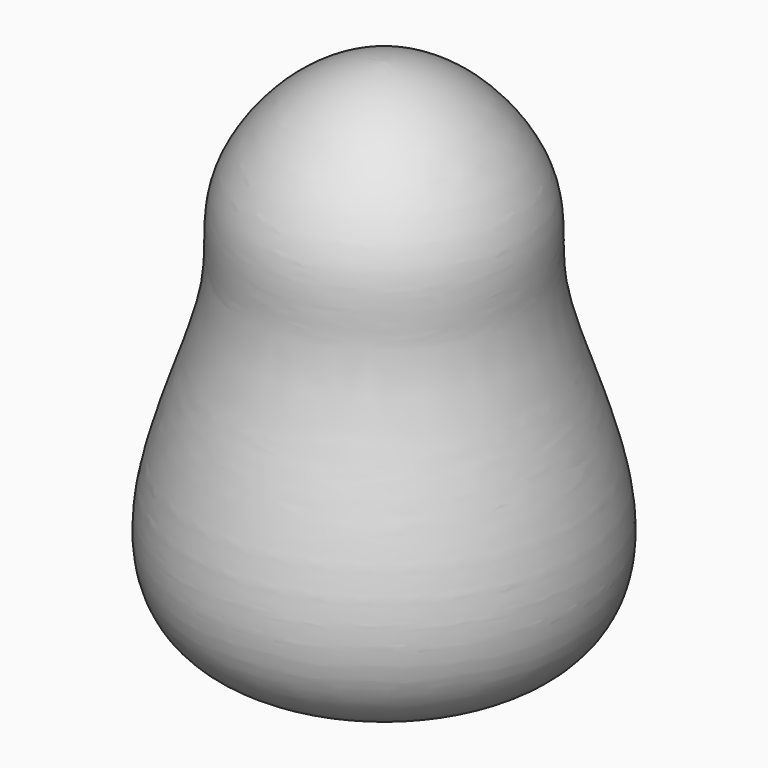
from build123d import *


with BuildPart() as f1:
    # F0 (on Front) → F1 (revolve)
    with BuildSketch(Plane.XZ):
        with BuildLine():
            Line((0, -52.3537062109), (0, 53.7330806255))
            add(Edge.make_bspline(
                [(0, 53.7330806255), (-13.1370157052, 53.3273076159), (-31.8709778241, 33.0857424774), (-25.4147994701, 12.1488706254), (-48.4003754541, -31.9097866922), (-32.2527586063, -56.3373678785), (0, -52.3537062109)],
                knots=[0, 0, 0, 0, 0.2460000401, 0.4374901801, 0.7136574986, 1, 1, 1, 1], degree=3))
        make_face()
    revolve(axis=Axis((0, 0, 0.6896872073), (0, 0, -1)))


solid = f1.part
